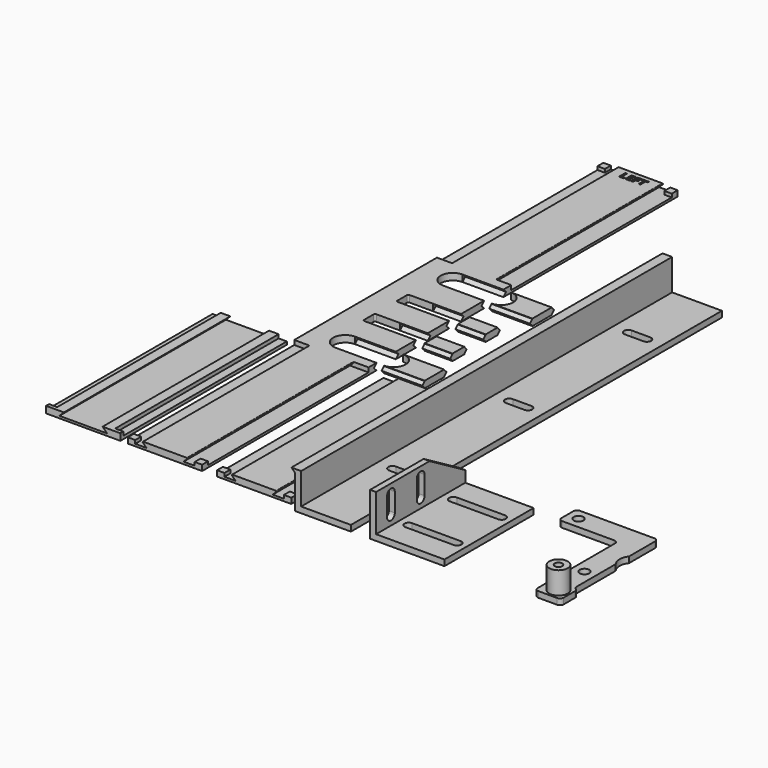
from build123d import *

# Parameters (mm, degrees)
F1_DEPTH      = 2.286
F0_W          = 25.4
F0_H          = 71.12
F0_W_2        = 9.525
F0_H_2        = 5.08
F0_H_3        = 5.0376876555
F3_DEPTH      = 71.12
F5_DEPTH      = 71.12
F6_W          = 2.54
F6_H          = 2.54
F7_DEPTH      = 1.143
F8_W          = 2.794
F8_H          = 69.85
F9_DEPTH      = 1.27
F11_DEPTH     = 13.97
F13_DEPTH     = 13.97
F16_DEPTH     = 9.525
F17_DEPTH     = 9.525
F18_TEXT_SIZE = 3.7573484911
F19_DEPTH     = 0.381
F21_DEPTH     = 158.5214
F23_DEPTH     = 158.5214
F25_DEPTH     = 2.032
F26_W         = 25.4
F26_H         = 38.1
F27_DEPTH     = 2.032
F28_W         = 2.032
F28_H         = 38.1
F29_DEPTH     = 12.7
F31_DEPTH     = 2.032
F32_R         = 1.2954
F32_R_2       = 1.651
F33_DEPTH     = 2.032
F34_R         = 3.175
F34_R_2       = 1.2954
F35_DEPTH     = 7.62


# Not quite as in the source:
# - Text() gives the source's letters only with a copy of the font that has no kerning and outlines rounded to 1/6400 em; it was checked with that copy


with BuildPart() as f1:
    # F0 (on Top) → F1 (new body)
    with BuildSketch(Plane.XY):
        with BuildLine():
            Line((-2.54, 131.2672), (-2.54, 205.74))
            Line((-2.54, 205.74), (-27.94, 205.74))
            Line((-27.94, 205.74), (-27.94, 2.54))
            Line((-27.94, 2.54), (-2.54, 2.54))
            Line((-2.54, 2.54), (-2.54, 77.0382))
            Line((-2.54, 77.0382), (-16.51, 77.0382))
            ThreePointArc((-16.51, 77.0382), (-20.6375, 81.1657), (-16.51, 85.2932))
            Line((-16.51, 85.2932), (-2.54, 85.2932))
            Line((-2.54, 85.2932), (-2.54, 93.8657))
            Line((-2.54, 93.8657), (-20.1295, 93.8657))
            ThreePointArc((-20.1295, 93.8657), (-20.4887102448, 94.0144897552), (-20.6375, 94.3737))
            Line((-20.6375, 94.3737), (-20.6375, 98.4377))
            ThreePointArc((-20.6375, 98.4377), (-20.4887102448, 98.7969102448), (-20.1295, 98.9457))
            Line((-20.1295, 98.9457), (-2.54, 98.9457))
            Line((-2.54, 98.9457), (-2.54, 108.0897))
            Line((-2.54, 108.0897), (-20.1295, 108.0897))
            ThreePointArc((-20.1295, 108.0897), (-20.4887102448, 108.2384897552), (-20.6375, 108.5977))
            Line((-20.6375, 108.5977), (-20.6375, 112.6617))
            ThreePointArc((-20.6375, 112.6617), (-20.4887102448, 113.0209102448), (-20.1295, 113.1697))
            Line((-20.1295, 113.1697), (-2.54, 113.1697))
            Line((-2.54, 113.1697), (-2.54, 123.0122))
            Line((-2.54, 123.0122), (-16.51, 123.0122))
            ThreePointArc((-16.51, 123.0122), (-20.6375, 127.1397), (-16.51, 131.2672))
            Line((-16.51, 131.2672), (-2.54, 131.2672))
        make_face()
    extrude(amount=F1_DEPTH)


with BuildPart() as f1b:
    # F0 (on Top) → F1, piece 2 (new body)
    with BuildSketch(Plane.XY):
        with Locations((-43.18, 38.1)):
            Rectangle(F0_W, F0_H)
    extrude(amount=F1_DEPTH)


with BuildPart() as f1c:
    # F0 (on Top) → F1, piece 3 (new body)
    with BuildSketch(Plane.XY):
        with Locations((15.24, 38.1)):
            Rectangle(F0_W, F0_H)
    extrude(amount=F1_DEPTH)


with BuildPart() as f1d:
    # F0 (on Top) → F1, piece 4 (new body)
    with BuildSketch(Plane.XY):
        with BuildLine():
            ThreePointArc((0, 85.2932), (4.1275, 81.1657), (0, 77.0382))
            Line((0, 77.0382), (13.97, 77.0382))
            Line((13.97, 77.0382), (13.97, 85.2932))
            Line((13.97, 85.2932), (0, 85.2932))
        make_face()
    extrude(amount=F1_DEPTH)

    # F12 (on face) → F13 (join)
    with BuildSketch(Plane.YZ.offset(13.97)):
        Polygon((77.0382, 0.127), (77.0382, 2.159), (76.0222, 1.143), align=None)
        Polygon((85.2932, 2.159), (85.2932, 0.127), (86.3092, 1.143), align=None)
    extrude(amount=-F13_DEPTH)


with BuildPart() as f1e:
    # F0 (on Top) → F1, piece 5 (new body)
    with BuildSketch(Plane.XY):
        with BuildLine():
            ThreePointArc((0, 131.2672), (4.1275, 127.1397), (0, 123.0122))
            Line((0, 123.0122), (13.97, 123.0122))
            Line((13.97, 123.0122), (13.97, 131.2672))
            Line((13.97, 131.2672), (0, 131.2672))
        make_face()
    extrude(amount=F1_DEPTH)

    # F12 (on face) → F13, piece 2 (join)
    with BuildSketch(Plane.YZ.offset(13.97)):
        Polygon((123.0122, 0.127), (123.0122, 2.159), (121.9962, 1.143), align=None)
        Polygon((131.2672, 2.159), (131.2672, 0.127), (132.2832, 1.143), align=None)
    extrude(amount=-F13_DEPTH)


with BuildPart() as f1f:
    # F0 (on Top) → F1, piece 6 (new body)
    with BuildSketch(Plane.XY):
        with Locations((5.1854069075, 110.6297)):
            Rectangle(F0_W_2, F0_H_2)
    extrude(amount=F1_DEPTH)

    # F14 (on face) → F17, piece 2 (join)
    with BuildSketch(Plane.YZ.offset(9.9479069075)):
        Polygon((108.0897, 0.127), (108.0897, 2.159), (107.0737, 1.143), align=None)
        Polygon((114.1857, 1.143), (113.1697, 2.159), (113.1697, 0.127), align=None)
    extrude(amount=-F17_DEPTH)


with BuildPart() as f1g:
    # F0 (on Top) → F1, piece 7 (new body)
    with BuildSketch(Plane.XY):
        with Locations((5.1854069075, 96.4268561723)):
            Rectangle(F0_W_2, F0_H_3)
    extrude(amount=F1_DEPTH)

    # F14 (on face) → F17 (join)
    with BuildSketch(Plane.YZ.offset(9.9479069075)):
        Polygon((93.9080123445, 0.127), (93.9080123445, 2.159), (92.8920123445, 1.143), align=None)
        Polygon((99.9617, 1.143), (98.9457, 2.159), (98.9457, 0.127), align=None)
    extrude(amount=-F17_DEPTH)


with BuildPart() as f3_tool:
    # F2 (on face) → F3 (new body)
    with BuildSketch(Plane.XZ.offset(-2.54)):
        with BuildLine():
            Line((-21.59, 0.762), (-22.8104764143, 1.9824764143))
            ThreePointArc((-22.8104764143, 1.9824764143), (-22.8490186095, 2.1762411143), (-22.6847528286, 2.286))
            Line((-22.6847528286, 2.286), (-27.94, 2.286))
            Line((-27.94, 2.286), (-27.94, 0.762))
            Line((-27.94, 0.762), (-21.59, 0.762))
        make_face()
        with BuildLine():
            Line((-7.6695235857, 1.9824764143), (-8.89, 0.762))
            Line((-8.89, 0.762), (-2.54, 0.762))
            Line((-2.54, 0.762), (-2.54, 2.286))
            Line((-2.54, 2.286), (-7.7952471714, 2.286))
            ThreePointArc((-7.7952471714, 2.286), (-7.6309813905, 2.1762411143), (-7.6695235857, 1.9824764143))
        make_face()
        Polygon((-36.576, 2.286), (-49.784, 2.286), (-51.308, 0.762), (-35.052, 0.762), align=None)
        with BuildLine():
            Line((7.7952471714, 2.286), (2.54, 2.286))
            Line((2.54, 2.286), (2.54, 0.762))
            Line((2.54, 0.762), (8.89, 0.762))
            Line((8.89, 0.762), (7.6695235857, 1.9824764143))
            ThreePointArc((7.6695235857, 1.9824764143), (7.6309813905, 2.1762411143), (7.7952471714, 2.286))
        make_face()
        with BuildLine():
            Line((21.59, 0.762), (27.94, 0.762))
            Line((27.94, 0.762), (27.94, 2.286))
            Line((27.94, 2.286), (22.6847528286, 2.286))
            ThreePointArc((22.6847528286, 2.286), (22.8490186095, 2.1762411143), (22.8104764143, 1.9824764143))
            Line((22.8104764143, 1.9824764143), (21.59, 0.762))
        make_face()
    extrude(amount=-F3_DEPTH)


with BuildPart() as f1_1:
    add(f1.part)

    # F3: cut by f3_tool
    add(f3_tool.part, mode=Mode.SUBTRACT)

    # F4 (on face) → F5 (cut)
    with BuildSketch(Plane(origin=(0, 205.74, 0), x_dir=(-1, 0, 0), z_dir=(0, 1, 0))):
        with BuildLine():
            Line((8.89, 0.762), (7.6695235857, 1.9824764143))
            ThreePointArc((7.6695235857, 1.9824764143), (7.6309813905, 2.1762411143), (7.7952471714, 2.286))
            Line((7.7952471714, 2.286), (2.54, 2.286))
            Line((2.54, 2.286), (2.54, 0.762))
            Line((2.54, 0.762), (8.89, 0.762))
        make_face()
        with BuildLine():
            Line((22.8104764143, 1.9824764143), (21.59, 0.762))
            Line((21.59, 0.762), (27.94, 0.762))
            Line((27.94, 0.762), (27.94, 2.286))
            Line((27.94, 2.286), (22.6847528286, 2.286))
            ThreePointArc((22.6847528286, 2.286), (22.8490186095, 2.1762411143), (22.8104764143, 1.9824764143))
        make_face()
    extrude(amount=-F5_DEPTH, mode=Mode.SUBTRACT)

    # F6 (on face) → F7, piece 2 (join)
    with BuildSketch(Plane.XY.offset(0.762)):
        with Locations((-3.81, 3.81)):
            Rectangle(F6_W, F6_H)
        with Locations((-26.67, 3.81)):
            Rectangle(F6_W, F6_H)
        with Locations((-26.67, 204.47)):
            Rectangle(F6_W, F6_H)
        with Locations((-3.81, 204.47)):
            Rectangle(F6_W, F6_H)
    extrude(amount=F7_DEPTH)

    # F10 (on face) → F11 (cut)
    with BuildSketch(Plane.YZ.offset(-2.54)):
        Polygon((86.4362, 1.143), (85.2932, 2.286), (85.2932, 0), align=None)
        Polygon((123.0122, 0), (123.0122, 2.286), (121.8692, 1.143), align=None)
        Polygon((132.4102, 1.143), (131.2672, 2.286), (131.2672, 0), align=None)
        Polygon((77.0382, 0), (77.0382, 2.286), (75.8952, 1.143), align=None)
    extrude(amount=-F11_DEPTH, mode=Mode.SUBTRACT)

    # F15 (on face) → F16 (cut)
    with BuildSketch(Plane.YZ.offset(-2.54)):
        Polygon((93.8657, 0), (93.8657, 2.286), (92.7227, 1.143), align=None)
        Polygon((100.0887, 1.143), (98.9457, 2.286), (98.9457, 0), align=None)
        Polygon((114.3127, 1.143), (113.1697, 2.286), (113.1697, 0), align=None)
        Polygon((108.0897, 0), (108.0897, 2.286), (106.9467, 1.143), align=None)
    extrude(amount=-F16_DEPTH, mode=Mode.SUBTRACT)

    # F18 (on face) → F19 (cut)
    with BuildSketch(Plane.XY.offset(2.286)):
        with Locations((-19.5531295011, 201.5107090864)):
            Text('LEFT', F18_TEXT_SIZE, font='Open Sans', font_style=FontStyle.BOLD, text_align=(TextAlign.LEFT, TextAlign.BOTTOM))
    extrude(amount=-F19_DEPTH, mode=Mode.SUBTRACT)


with BuildPart() as f1b_1:
    add(f1b.part)

    # F3: cut by f3_tool
    add(f3_tool.part, mode=Mode.SUBTRACT)

    # F8 (on face) → F9 (cut)
    with BuildSketch(Plane.XY.offset(2.286)):
        with Locations((-31.877, 38.735)):
            Rectangle(F8_W, F8_H)
        with Locations((-54.483, 38.735)):
            Rectangle(F8_W, F8_H)
    extrude(amount=-F9_DEPTH, mode=Mode.SUBTRACT)


with BuildPart() as f1c_1:
    add(f1c.part)

    # F3: cut by f3_tool
    add(f3_tool.part, mode=Mode.SUBTRACT)

    # F6 (on face) → F7 (join)
    with BuildSketch(Plane.XY.offset(0.762)):
        with Locations((26.67, 3.81)):
            Rectangle(F6_W, F6_H)
        with Locations((3.81, 3.81)):
            Rectangle(F6_W, F6_H)
    extrude(amount=F7_DEPTH)


with BuildPart() as f21:
    # F20 (on Front) → F21 (new body)
    with BuildSketch(Plane.XZ):
        Polygon((33.3323611147, 12.7), (31.3003611147, 12.7), (31.3003611147, 0), (50.3503611147, 0), (50.3503611147, 2.032), (33.3323611147, 2.032), align=None)
    extrude(amount=-F21_DEPTH)

    # F22 (on face) → F23 (join)
    with BuildSketch(Plane.XZ):
        Polygon((31.3003611147, 11.43), (31.3003611147, 12.7), (30.0303611147, 12.7), align=None)
    extrude(amount=-F23_DEPTH)

    # F24 (on face) → F25 (cut, through all)
    with BuildSketch(Plane.XY.offset(2.032)):
        with BuildLine():
            Line((38.6663611147, 30.9245), (45.0163611147, 30.9245))
            ThreePointArc((45.0163611147, 30.9245), (46.4768611147, 32.385), (45.0163611147, 33.8455))
            Line((45.0163611147, 33.8455), (38.6663611147, 33.8455))
            ThreePointArc((38.6663611147, 33.8455), (37.2058611147, 32.385), (38.6663611147, 30.9245))
        make_face()
        with BuildLine():
            Line((38.6663611147, 131.6609), (45.0163611147, 131.6609))
            ThreePointArc((45.0163611147, 131.6609), (46.4768611147, 133.1214), (45.0163611147, 134.5819))
            Line((45.0163611147, 134.5819), (38.6663611147, 134.5819))
            ThreePointArc((38.6663611147, 134.5819), (37.2058611147, 133.1214), (38.6663611147, 131.6609))
        make_face()
        with BuildLine():
            Line((38.6663611147, 80.8609), (45.0163611147, 80.8609))
            ThreePointArc((45.0163611147, 80.8609), (46.4768611147, 82.3214), (45.0163611147, 83.7819))
            Line((45.0163611147, 83.7819), (38.6663611147, 83.7819))
            ThreePointArc((38.6663611147, 83.7819), (37.2058611147, 82.3214), (38.6663611147, 80.8609))
        make_face()
    extrude(amount=-F25_DEPTH, mode=Mode.SUBTRACT)


with BuildPart() as f27:
    # F26 (on Top) → F27 (new body)
    with BuildSketch(Plane.XY):
        with Locations((69.6213900466, 19.05)):
            Rectangle(F26_W, F26_H)
        with BuildLine():
            ThreePointArc((62.5093900466, 8.0645), (61.0488900466, 9.525), (62.5093900466, 10.9855))
            Line((62.5093900466, 10.9855), (79.0193900466, 10.9855))
            ThreePointArc((79.0193900466, 10.9855), (80.4798900466, 9.525), (79.0193900466, 8.0645))
            Line((79.0193900466, 8.0645), (62.5093900466, 8.0645))
        make_face(mode=Mode.SUBTRACT)
        with BuildLine():
            ThreePointArc((62.5093900466, 27.1145), (61.0488900466, 28.575), (62.5093900466, 30.0355))
            Line((62.5093900466, 30.0355), (79.0193900466, 30.0355))
            ThreePointArc((79.0193900466, 30.0355), (80.4798900466, 28.575), (79.0193900466, 27.1145))
            Line((79.0193900466, 27.1145), (62.5093900466, 27.1145))
        make_face(mode=Mode.SUBTRACT)
    extrude(amount=F27_DEPTH)

    # F28 (on face) → F29 (join)
    with BuildSketch(Plane.XY.offset(2.032)):
        with Locations((57.9373900466, 19.05)):
            Rectangle(F28_W, F28_H)
    extrude(amount=F29_DEPTH)

    # F30 (on face) → F31 (cut, through all)
    with BuildSketch(Plane.YZ.offset(58.9533900466)):
        with BuildLine():
            Line((8.001, 5.207), (8.001, 11.557))
            ThreePointArc((8.001, 11.557), (6.35, 13.208), (4.699, 11.557))
            Line((4.699, 11.557), (4.699, 5.207))
            ThreePointArc((4.699, 5.207), (6.35, 3.556), (8.001, 5.207))
        make_face()
        with BuildLine():
            Line((20.701, 5.207), (20.701, 11.557))
            ThreePointArc((20.701, 11.557), (19.05, 13.208), (17.399, 11.557))
            Line((17.399, 11.557), (17.399, 5.207))
            ThreePointArc((17.399, 5.207), (19.05, 3.556), (20.701, 5.207))
        make_face()
        Polygon((38.1, 14.732), (22.86, 14.732), (38.1, 5.842), align=None)
    extrude(amount=-F31_DEPTH, mode=Mode.SUBTRACT)


with BuildPart() as f33:
    # F32 (on Top) → F33 (new body)
    with BuildSketch(Plane.XY):
        with BuildLine():
            Line((112.0778166699, 35.6627096211), (112.0778166699, 2.6427096211))
            ThreePointArc((112.0778166699, 2.6427096211), (112.4497910578, 1.744684009), (113.3478166699, 1.3727096211))
            Line((113.3478166699, 1.3727096211), (119.6978166699, 1.3727096211))
            ThreePointArc((119.6978166699, 1.3727096211), (120.595842282, 1.744684009), (120.9678166699, 2.6427096211))
            Line((120.9678166699, 2.6427096211), (120.9678166699, 7.5146074779))
            ThreePointArc((120.9678166699, 7.5146074779), (120.8019219925, 8.1421833193), (120.347578187, 8.6058040555))
            Line((120.347578187, 8.6058040555), (120.3180551529, 8.6233837765))
            ThreePointArc((120.3180551529, 8.6233837765), (119.8637113474, 9.0870045128), (119.6978166699, 9.7145803541))
            Line((119.6978166699, 9.7145803541), (119.6978166699, 26.4552096211))
            ThreePointArc((119.6978166699, 26.4552096211), (118.7453166699, 29.3127096211), (119.6978166699, 32.1702096211))
            Line((119.6978166699, 32.1702096211), (119.6978166699, 43.2827096211))
            ThreePointArc((119.6978166699, 43.2827096211), (119.325842282, 44.1807352332), (118.4278166699, 44.5527096211))
            Line((118.4278166699, 44.5527096211), (93.0278166699, 44.5527096211))
            ThreePointArc((93.0278166699, 44.5527096211), (92.1297910578, 44.1807352332), (91.7578166699, 43.2827096211))
            Line((91.7578166699, 43.2827096211), (91.7578166699, 38.2027096211))
            ThreePointArc((91.7578166699, 38.2027096211), (92.1297910578, 37.304684009), (93.0278166699, 36.9327096211))
            Line((93.0278166699, 36.9327096211), (110.8078166699, 36.9327096211))
            ThreePointArc((110.8078166699, 36.9327096211), (111.705842282, 36.5607352332), (112.0778166699, 35.6627096211))
        make_face()
        with Locations((117.1578166699, 5.1827096211)):
            Circle(F32_R, mode=Mode.SUBTRACT)
        with Locations((115.8878166699, 17.8827096211)):
            Circle(F32_R_2, mode=Mode.SUBTRACT)
        with Locations((95.5678166699, 40.7427096211)):
            Circle(F32_R_2, mode=Mode.SUBTRACT)
    extrude(amount=F33_DEPTH)

    # F34 (on face) → F35 (join)
    with BuildSketch(Plane.XY.offset(2.032)):
        with Locations((117.1578166699, 5.1827096211)):
            Circle(F34_R)
        with Locations((117.1578166699, 5.1827096211)):
            Circle(F34_R_2, mode=Mode.SUBTRACT)
    extrude(amount=F35_DEPTH)


solid = Compound([f1d.part, f1e.part, f1f.part, f1g.part, f1_1.part, f1b_1.part, f1c_1.part, f21.part, f27.part, f33.part])
